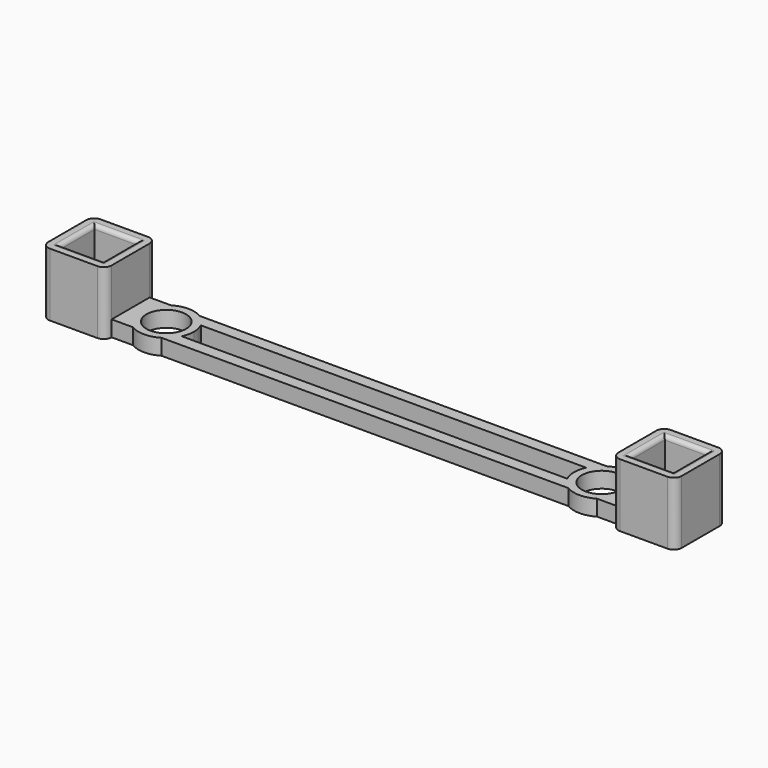
from build123d import *

# Parameters (mm, degrees)
F0_R          = 1.25
F1_DEPTH      = 1
F2_W          = 4
F2_H          = 4
F2_W_2        = 2.7
F2_H_2        = 2.7
F3_DEPTH      = 3
F3_DEPTH_BACK = 1
F4_R          = 0.49999
F5_R          = 0.25


# Not quite as in the source:
# - a fillet or chamfer is up to 0.001 mm smaller than in the source, because OpenCascade refuses the exact size


with BuildPart() as f1:
    # F0 (on Top) → F1 (new body)
    with BuildSketch(Plane.XY):
        with BuildLine():
            Line((0, 0.75), (0, 1.5))
            Line((0, 1.5), (-12.8486121811, 1.5))
            ThreePointArc((-12.8486121811, 1.5), (-12.4533274736, 1.1752192814), (-12.1688611699, 0.75))
            Line((-12.1688611699, 0.75), (0, 0.75))
        make_face()
        with BuildLine():
            ThreePointArc((-12.1688611699, 0.75), (-12.4533274736, 1.1752192814), (-12.8486121811, 1.5))
            Line((-12.8486121811, 1.5), (-14.6513878189, 1.5))
            ThreePointArc((-14.6513878189, 1.5), (-15.5, 0), (-14.6513878189, -1.5))
            Line((-14.6513878189, -1.5), (-12.8486121811, -1.5))
            ThreePointArc((-12.8486121811, -1.5), (-12.4533274736, -1.1752192814), (-12.1688611699, -0.75))
            ThreePointArc((-12.1688611699, -0.75), (-12.0427371391, -0.3843872054), (-12, 0))
            ThreePointArc((-12, 0), (-12.0427371391, 0.3843872054), (-12.1688611699, 0.75))
        make_face()
        with Locations((-13.75, 0)):
            Circle(F0_R, mode=Mode.SUBTRACT)
        with BuildLine():
            Line((-14.6513878189, 1.5), (-12.8486121811, 1.5))
            ThreePointArc((-12.8486121811, 1.5), (-13.75, 1.75), (-14.6513878189, 1.5))
        make_face()
        with BuildLine():
            ThreePointArc((-14.6513878189, -1.5), (-15.5, 0), (-14.6513878189, 1.5))
            Line((-14.6513878189, 1.5), (-19.5, 1.5))
            Line((-19.5, 1.5), (-19.5, -1.5))
            Line((-19.5, -1.5), (-14.6513878189, -1.5))
        make_face()
        with BuildLine():
            Line((-12.8486121811, -1.5), (-14.6513878189, -1.5))
            ThreePointArc((-14.6513878189, -1.5), (-13.75, -1.75), (-12.8486121811, -1.5))
        make_face()
        with BuildLine():
            ThreePointArc((-12.1688611699, -0.75), (-12.4533274736, -1.1752192814), (-12.8486121811, -1.5))
            Line((-12.8486121811, -1.5), (0, -1.5))
            Line((0, -1.5), (0, -0.75))
            Line((0, -0.75), (-12.1688611699, -0.75))
        make_face()
    extrude(amount=F1_DEPTH)

    # F2 (on face) → F3 (join, two sides)
    with BuildSketch(Plane.XY.offset(1)) as f3_sk:
        with Locations((-18, 0)):
            Rectangle(F2_W, F2_H)
        with Locations((-18, 0)):
            Rectangle(F2_W_2, F2_H_2, mode=Mode.SUBTRACT)
    extrude(amount=F3_DEPTH)
    extrude(f3_sk.sketch, amount=-F3_DEPTH_BACK)

    # F4 (radius 0.5 in the source; OpenCascade refuses exactly that, so slightly less here)
    f4_edges = [f1.edges().sort_by_distance(p)[0] for p in [
        (-16, -2, 2),
        (-20, -2, 2),
        (-16, 2, 2),
        (-20, 2, 2),
    ]]
    fillet(f4_edges, radius=F4_R)

    # F5
    f5_edges = [f1.edges().sort_by_distance(p)[0] for p in [
        (-18, -1.35, 4),
        (-16.65, 0, 4),
        (-18, 1.35, 4),
        (-19.35, 0, 4),
    ]]
    fillet(f5_edges, radius=F5_R)

    # F6: F1 across plane


with BuildPart() as f1_1:
    add(f1.part)
    add(f1.part.mirror(Plane.YZ))


solid = f1_1.part
